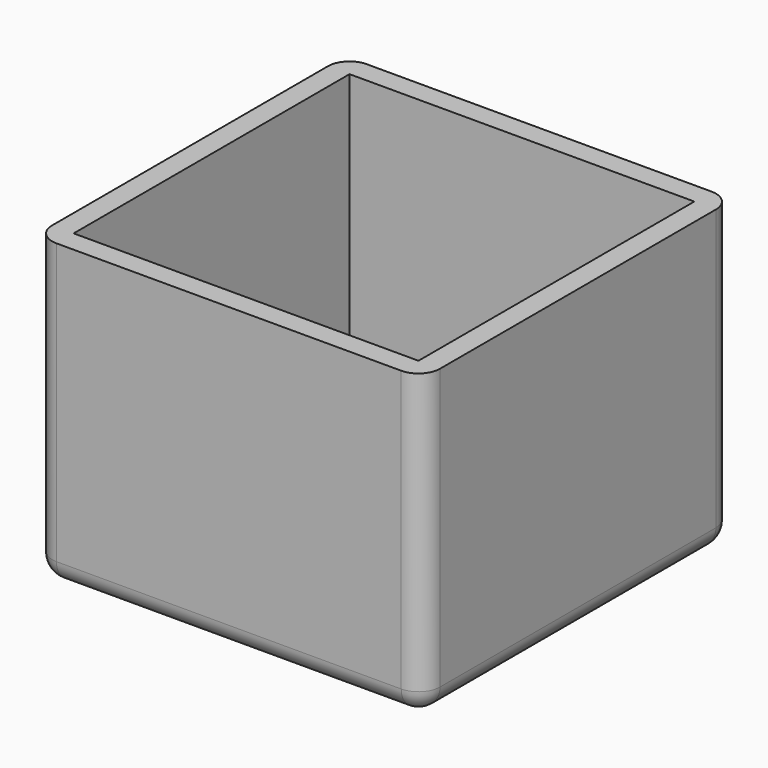
from build123d import *

# Parameters (mm, degrees)
F0_W         = 91.44
F0_H         = 91.44
F0_W_2       = 81.28
F0_H_2       = 81.28
F1_DEPTH     = 71.12
F2_DEPTH     = 5.08
F3_R         = 5.08
F4_TEXT_SIZE = 11.0066651056
F5_DEPTH     = 1.27


# Not quite as in the source:
# - Text() gives the source's letters only with a copy of the font that has no kerning and outlines rounded to 1/6400 em; it was checked with that copy


with BuildPart() as f1:
    # F0 (on Top) → F1 (new body)
    with BuildSketch(Plane.XY):
        with Locations((16.4591988486, 15.0875956277)):
            Rectangle(F0_W, F0_H)
        with Locations((16.4591988486, 15.0875956277)):
            Rectangle(F0_W_2, F0_H_2, mode=Mode.SUBTRACT)
    extrude(amount=F1_DEPTH)

    # F0 (on Top) → F2 (join)
    with BuildSketch(Plane.XY):
        with Locations((16.4591988486, 15.0875956277)):
            Rectangle(F0_W_2, F0_H_2)
    extrude(amount=F2_DEPTH)

    # F3
    f3_edges = [f1.edges().sort_by_distance(p)[0] for p in [
        (62.179199, 60.807596, 35.56),
        (-29.260801, 60.807596, 35.56),
        (-29.260801, -30.632404, 35.56),
        (62.179199, -30.632404, 35.56),
        (62.179199, 15.087596, 0),
        (16.459199, -30.632404, 0),
        (-29.260801, 15.087596, 0),
        (16.459199, 60.807596, 0),
    ]]
    fillet(f3_edges, radius=F3_R)

    # F4 (on face) → F5 (cut)
    with BuildSketch(Plane(origin=(0, 0, 0), x_dir=(1, 0, 0), z_dir=(0, 0, -1))):
        with Locations((-19.5072013885, 13.2587999105)):
            Text('Benjamin', F4_TEXT_SIZE, font='Open Sans', font_style=FontStyle.BOLD, text_align=(TextAlign.LEFT, TextAlign.BOTTOM))
        with Locations((-19.5072013885, -1.7102646331)):
            Text('Child', F4_TEXT_SIZE, font='Open Sans', font_style=FontStyle.BOLD, text_align=(TextAlign.LEFT, TextAlign.BOTTOM))
    extrude(amount=-F5_DEPTH, mode=Mode.SUBTRACT)


solid = f1.part
